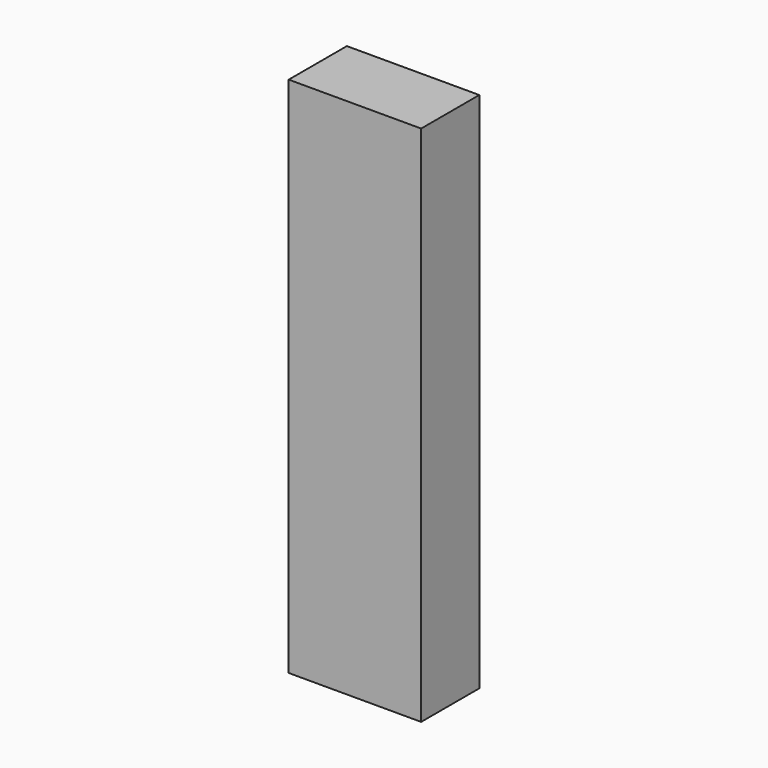
from build123d import *

# Parameters (mm, degrees)
F2_W     = 2.3150034249
F2_H     = 9.1314045712
F3_DEPTH = 1.27


# Not quite as in the source:
# - the program builds the solid bodies; features that only make, move or delete a surface that nothing else refers to are left out


with BuildPart() as f3:
    # F2 (on Front) → F3 (new body)
    with BuildSketch(Plane.XZ):
        with Locations((-0.0635847682, -0.2150074579)):
            Rectangle(F2_W, F2_H)
    extrude(amount=-F3_DEPTH)


solid = f3.part
